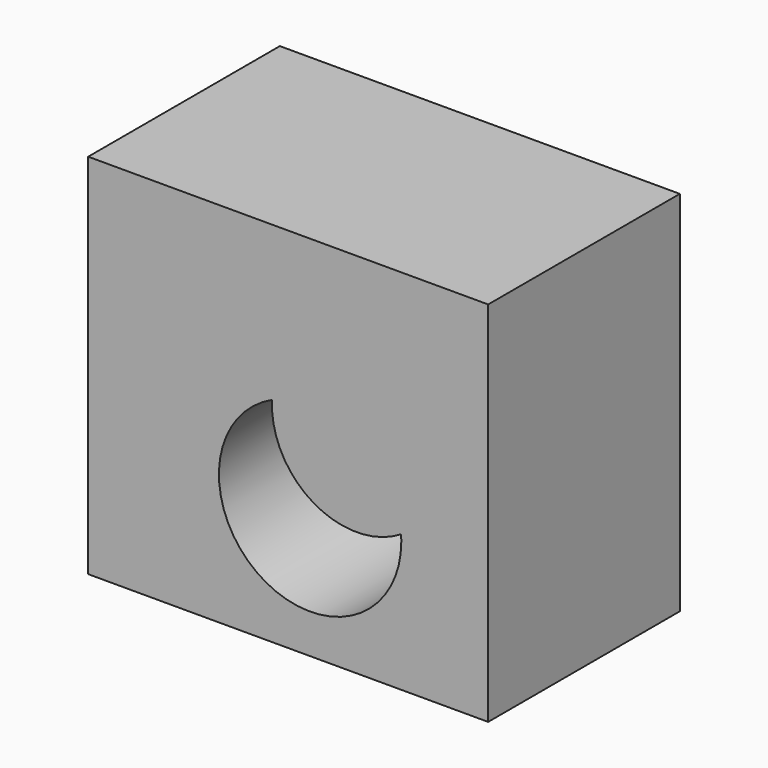
from build123d import *

# Parameters (mm, degrees)
F0_W     = 42.4149371684
F0_H     = 38.9721691608
F1_DEPTH = 25.4
F5_DEPTH = 25


# Not quite as in the source:
# - the program builds the solid bodies; features that only make, move or delete a surface that nothing else refers to are left out


with BuildPart() as f1:
    # F0 (on Front) → F1 (new body)
    with BuildSketch(Plane.XZ):
        with Locations((21.2074685842, 19.4860845804)):
            Rectangle(F0_W, F0_H)
    extrude(amount=F1_DEPTH)

    # F4 (on face) → F5 (cut)
    with BuildSketch(Plane.XZ.offset(25.4)):
        with BuildLine():
            ThreePointArc((19.4994620307, 22.614925386), (18.3126908163, 5.6894142875), (33.200540329, 13.8277979568))
            ThreePointArc((33.200540329, 13.8277979568), (33.1944083659, 14.1720857887), (33.176020255, 14.5159369041))
            ThreePointArc((33.176020255, 14.5159369041), (23.8873414039, 14.4275027139), (19.4994620307, 22.614925386))
        make_face()
    extrude(amount=-F5_DEPTH, mode=Mode.SUBTRACT)


solid = f1.part
